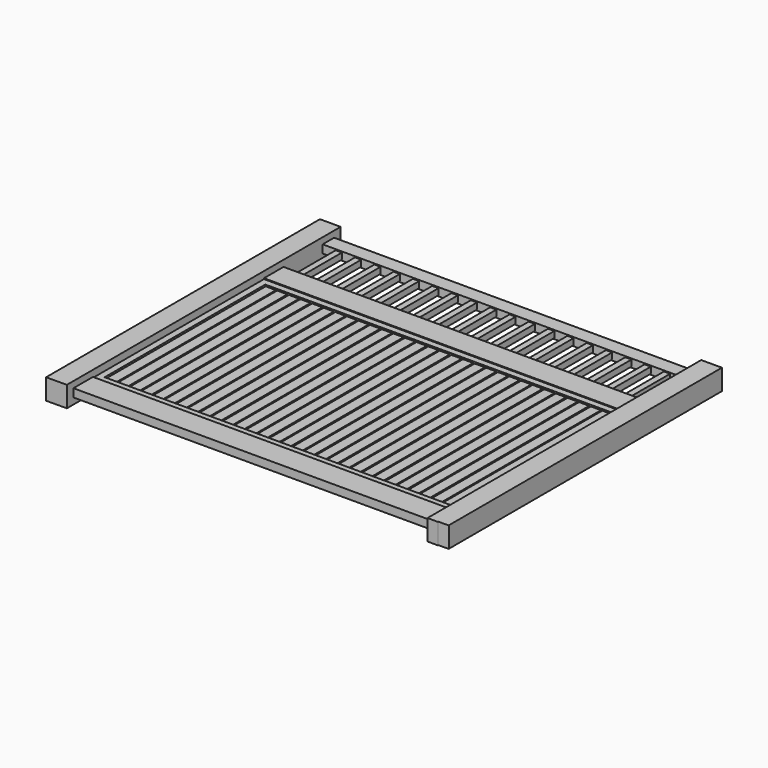
from build123d import *

# Parameters (mm, degrees)
F1_DEPTH      = 63.5
F1_DEPTH_BACK = 63.5
F2_DEPTH      = 25
F2_DEPTH_BACK = 25
F0_W          = 2213
F0_H          = 150
F0_W_2        = 40
F0_H_2        = 1232
F3_DEPTH      = 20
F3_DEPTH_BACK = 20
F0_W_3        = 38
F0_H_3        = 300
F4_DEPTH      = 19
F4_DEPTH_BACK = 19
F6_DEPTH      = 825
F6_DEPTH_BACK = 487.5


with BuildPart() as f1:
    # F0 (on Top) → F1 (new body, two sides)
    with BuildSketch(Plane.XY) as f1_sk:
        Polygon((1106.5, -1050), (1170, -1050), (1170, -1047.6227045059), align=None)
        Polygon((1106.5, -1000), (1106.5, -1050), (1170, -1047.6227045059), (1233.5, -1045.2454090118), (1233.5, 1050), (1170, 1050), (1106.5, 1050), (1106.5, 1000), (1106.5, 912), (1106.5, 612), (1106.5, 462), (1106.5, 422), (1106.5, -810), (1106.5, -850), align=None)
    extrude(amount=F1_DEPTH)
    extrude(f1_sk.sketch, amount=-F1_DEPTH_BACK)


with BuildPart() as f1b:
    # F0 (on Top) → F1, piece 2 (new body, two sides)
    with BuildSketch(Plane.XY) as f1_2_sk:
        Polygon((-1106.5, -1050), (-1106.5, -1000), (-1106.5, -850), (-1106.5, -810), (-1106.5, 422), (-1106.5, 462), (-1106.5, 612), (-1106.5, 912), (-1106.5, 1000), (-1106.5, 1050), (-1170, 1050), (-1233.5, 1050), (-1233.5, -1050.8052110672), align=None)
    extrude(amount=F1_DEPTH)
    extrude(f1_2_sk.sketch, amount=-F1_DEPTH_BACK)


with BuildPart() as f2:
    # F0 (on Top) → F2 (new body, two sides)
    with BuildSketch(Plane.XY) as f2_sk:
        Polygon((1106.5, 912), (1106.5, 1000), (-1106.5, 1000), (-1106.5, 912), (-1026.03, 912), (-988.03, 912), (-907.56, 912), (-869.56, 912), (-789.09, 912), (-751.09, 912), (-670.62, 912), (-632.62, 912), (-552.15, 912), (-514.15, 912), (-433.68, 912), (-395.68, 912), (-315.21, 912), (-277.21, 912), (-196.74, 912), (-158.74, 912), (-78.27, 912), (-40.27, 912), (40.2, 912), (78.2, 912), (158.67, 912), (196.67, 912), (277.14, 912), (315.14, 912), (395.61, 912), (433.61, 912), (514.08, 912), (552.08, 912), (632.55, 912), (670.55, 912), (751.02, 912), (789.02, 912), (869.49, 912), (907.49, 912), (987.96, 912), (1025.96, 912), align=None)
    extrude(amount=F2_DEPTH)
    extrude(f2_sk.sketch, amount=-F2_DEPTH_BACK)


with BuildPart() as f2b:
    # F0 (on Top) → F2, piece 2 (new body, two sides)
    with BuildSketch(Plane.XY) as f2_2_sk:
        Polygon((-1106.5, 462), (1106.5, 462), (1106.5, 612), (1025.96, 612), (987.96, 612), (907.49, 612), (869.49, 612), (789.02, 612), (751.02, 612), (670.55, 612), (632.55, 612), (552.08, 612), (514.08, 612), (433.61, 612), (395.61, 612), (315.14, 612), (277.14, 612), (196.67, 612), (158.67, 612), (78.2, 612), (40.2, 612), (-40.27, 612), (-78.27, 612), (-158.74, 612), (-196.74, 612), (-277.21, 612), (-315.21, 612), (-395.68, 612), (-433.68, 612), (-514.15, 612), (-552.15, 612), (-632.62, 612), (-670.62, 612), (-751.09, 612), (-789.09, 612), (-869.56, 612), (-907.56, 612), (-988.03, 612), (-1026.03, 612), (-1106.5, 612), align=None)
    extrude(amount=F2_DEPTH)
    extrude(f2_2_sk.sketch, amount=-F2_DEPTH_BACK)


with BuildPart() as f2c:
    # F0 (on Top) → F2, piece 3 (new body, two sides)
    with BuildSketch(Plane.XY) as f2_3_sk:
        with Locations((0, -925)):
            Rectangle(F0_W, F0_H)
    extrude(amount=F2_DEPTH)
    extrude(f2_3_sk.sketch, amount=-F2_DEPTH_BACK)


with BuildPart() as f3:
    # F0 (on Top) → F3 (new body, two sides)
    with BuildSketch(Plane.XY) as f3_sk:
        Polygon((1066.5, 422), (1106.5, 422), (1106.5, 462), (-1106.5, 462), (-1106.5, 422), (-1066.5, 422), align=None)
        with Locations((1086.5, -194)):
            Rectangle(F0_W_2, F0_H_2)
        Polygon((-1106.5, -850), (1106.5, -850), (1106.5, -810), (1066.5, -810), (-1066.5, -810), (-1106.5, -810), align=None)
        with Locations((-1086.5, -194)):
            Rectangle(F0_W_2, F0_H_2)
    extrude(amount=F3_DEPTH)
    extrude(f3_sk.sketch, amount=-F3_DEPTH_BACK)

    # F5 (on Front) → F6 (join, two sides)
    with BuildSketch(Plane.XZ) as f6_sk:
        Polygon((-992.4924378616, -11), (-931.2006182523, -11), (-927.5, -7.6376459808), (-927.5, 7.3770178367), (-930.9458671252, 11), (-993.3938319101, 11), (-997.3938319101, 8), (-1001.3938319101, 11), (-1063.7911305095, 11), (-1067.5, 7.6467497703), (-1067.5, -8.3163099906), (-1063.2812551709, -11), (-1000.4924378616, -11), (-996.4924378616, -8), align=None)
        Polygon((-920.7812551709, -11), (-857.9924378616, -11), (-853.9924378616, -8), (-849.9924378616, -11), (-788.7006182523, -11), (-785, -7.6376459808), (-785, 7.3770178367), (-788.4458671252, 11), (-850.8938319101, 11), (-854.8938319101, 8), (-858.8938319101, 11), (-921.2911305095, 11), (-925, 7.6467497703), (-925, -8.3163099906), align=None)
        Polygon((-778.2812551709, -11), (-715.4924378616, -11), (-711.4924378616, -8), (-707.4924378616, -11), (-646.2006182523, -11), (-642.5, -7.6376459808), (-642.5, 7.3770178367), (-645.9458671252, 11), (-708.3938319101, 11), (-712.3938319101, 8), (-716.3938319101, 11), (-778.7911305095, 11), (-782.5, 7.6467497703), (-782.5, -8.3163099906), align=None)
        Polygon((-635.7812551709, -11), (-572.9924378616, -11), (-568.9924378616, -8), (-564.9924378616, -11), (-503.7006182523, -11), (-500, -7.6376459808), (-500, 7.3770178367), (-503.4458671252, 11), (-565.8938319101, 11), (-569.8938319101, 8), (-573.8938319101, 11), (-636.2911305095, 11), (-640, 7.6467497703), (-640, -8.3163099906), align=None)
        Polygon((-493.2812551709, -11), (-430.4924378616, -11), (-426.4924378616, -8), (-422.4924378616, -11), (-361.2006182523, -11), (-357.5, -7.6376459808), (-357.5, 7.3770178367), (-360.9458671252, 11), (-423.3938319101, 11), (-427.3938319101, 8), (-431.3938319101, 11), (-493.7911305095, 11), (-497.5, 7.6467497703), (-497.5, -8.3163099906), align=None)
        Polygon((-350.7812551709, -11), (-287.9924378616, -11), (-283.9924378616, -8), (-279.9924378616, -11), (-218.7006182523, -11), (-215, -7.6376459808), (-215, 7.3770178367), (-218.4458671252, 11), (-280.8938319101, 11), (-284.8938319101, 8), (-288.8938319101, 11), (-351.2911305095, 11), (-355, 7.6467497703), (-355, -8.3163099906), align=None)
        Polygon((-208.2812551709, -11), (-145.4924378616, -11), (-141.4924378616, -8), (-137.4924378616, -11), (-76.2006182523, -11), (-72.5, -7.6376459808), (-72.5, 7.3770178367), (-75.9458671252, 11), (-138.3938319101, 11), (-142.3938319101, 8), (-146.3938319101, 11), (-208.7911305095, 11), (-212.5, 7.6467497703), (-212.5, -8.3163099906), align=None)
        Polygon((-65.7812551709, -11), (-2.9924378616, -11), (1.0075621384, -8), (5.0075621384, -11), (66.2993817477, -11), (70, -7.6376459808), (70, 7.3770178367), (66.5541328748, 11), (4.1061680899, 11), (0.1061680899, 8), (-3.8938319101, 11), (-66.2911305095, 11), (-70, 7.6467497703), (-70, -8.3163099906), align=None)
        Polygon((76.7187448291, -11), (139.5075621384, -11), (143.5075621384, -8), (147.5075621384, -11), (208.7993817477, -11), (212.5, -7.6376459808), (212.5, 7.3770178367), (209.0541328748, 11), (146.6061680899, 11), (142.6061680899, 8), (138.6061680899, 11), (76.2088694905, 11), (72.5, 7.6467497703), (72.5, -8.3163099906), align=None)
        Polygon((219.2187448291, -11), (282.0075621384, -11), (286.0075621384, -8), (290.0075621384, -11), (351.2993817477, -11), (355, -7.6376459808), (355, 7.3770178367), (351.5541328748, 11), (289.1061680899, 11), (285.1061680899, 8), (281.1061680899, 11), (218.7088694905, 11), (215, 7.6467497703), (215, -8.3163099906), align=None)
        Polygon((361.7187448291, -11), (424.5075621384, -11), (428.5075621384, -8), (432.5075621384, -11), (493.7993817477, -11), (497.5, -7.6376459808), (497.5, 7.3770178367), (494.0541328748, 11), (431.6061680899, 11), (427.6061680899, 8), (423.6061680899, 11), (361.2088694905, 11), (357.5, 7.6467497703), (357.5, -8.3163099906), align=None)
        Polygon((504.2187448291, -11), (567.0075621384, -11), (571.0075621384, -8), (575.0075621384, -11), (636.2993817477, -11), (640, -7.6376459808), (640, 7.3770178367), (636.5541328748, 11), (574.1061680899, 11), (570.1061680899, 8), (566.1061680899, 11), (503.7088694905, 11), (500, 7.6467497703), (500, -8.3163099906), align=None)
        Polygon((646.7187448291, -11), (709.5075621384, -11), (713.5075621384, -8), (717.5075621384, -11), (778.7993817477, -11), (782.5, -7.6376459808), (782.5, 7.3770178367), (779.0541328748, 11), (716.6061680899, 11), (712.6061680899, 8), (708.6061680899, 11), (646.2088694905, 11), (642.5, 7.6467497703), (642.5, -8.3163099906), align=None)
        Polygon((789.2187448291, -11), (852.0075621384, -11), (856.0075621384, -8), (860.0075621384, -11), (921.2993817477, -11), (925, -7.6376459808), (925, 7.3770178367), (921.5541328748, 11), (859.1061680899, 11), (855.1061680899, 8), (851.1061680899, 11), (788.7088694905, 11), (785, 7.6467497703), (785, -8.3163099906), align=None)
        Polygon((931.7187448291, -11), (994.5075621384, -11), (998.5075621384, -8), (1002.5075621384, -11), (1063.7993817477, -11), (1067.5, -7.6376459808), (1067.5, 7.3770178367), (1064.0541328748, 11), (1001.6061680899, 11), (997.6061680899, 8), (993.6061680899, 11), (931.2088694905, 11), (927.5, 7.6467497703), (927.5, -8.3163099906), align=None)
    extrude(amount=F6_DEPTH)
    extrude(f6_sk.sketch, amount=-F6_DEPTH_BACK)


with BuildPart() as f4:
    # F0 (on Top) → F4 (new body, two sides)
    with BuildSketch(Plane.XY) as f4_sk:
        with Locations((-1007.03, 762)):
            Rectangle(F0_W_3, F0_H_3)
    extrude(amount=F4_DEPTH)
    extrude(f4_sk.sketch, amount=-F4_DEPTH_BACK)


with BuildPart() as f4b:
    # F0 (on Top) → F4, piece 2 (new body, two sides)
    with BuildSketch(Plane.XY) as f4_2_sk:
        with Locations((-888.56, 762)):
            Rectangle(F0_W_3, F0_H_3)
    extrude(amount=F4_DEPTH)
    extrude(f4_2_sk.sketch, amount=-F4_DEPTH_BACK)


with BuildPart() as f4c:
    # F0 (on Top) → F4, piece 3 (new body, two sides)
    with BuildSketch(Plane.XY) as f4_3_sk:
        with Locations((-770.09, 762)):
            Rectangle(F0_W_3, F0_H_3)
    extrude(amount=F4_DEPTH)
    extrude(f4_3_sk.sketch, amount=-F4_DEPTH_BACK)


with BuildPart() as f4d:
    # F0 (on Top) → F4, piece 4 (new body, two sides)
    with BuildSketch(Plane.XY) as f4_4_sk:
        with Locations((-651.62, 762)):
            Rectangle(F0_W_3, F0_H_3)
    extrude(amount=F4_DEPTH)
    extrude(f4_4_sk.sketch, amount=-F4_DEPTH_BACK)


with BuildPart() as f4e:
    # F0 (on Top) → F4, piece 5 (new body, two sides)
    with BuildSketch(Plane.XY) as f4_5_sk:
        with Locations((-533.15, 762)):
            Rectangle(F0_W_3, F0_H_3)
    extrude(amount=F4_DEPTH)
    extrude(f4_5_sk.sketch, amount=-F4_DEPTH_BACK)


with BuildPart() as f4f:
    # F0 (on Top) → F4, piece 6 (new body, two sides)
    with BuildSketch(Plane.XY) as f4_6_sk:
        with Locations((-414.68, 762)):
            Rectangle(F0_W_3, F0_H_3)
    extrude(amount=F4_DEPTH)
    extrude(f4_6_sk.sketch, amount=-F4_DEPTH_BACK)


with BuildPart() as f4g:
    # F0 (on Top) → F4, piece 7 (new body, two sides)
    with BuildSketch(Plane.XY) as f4_7_sk:
        with Locations((-296.21, 762)):
            Rectangle(F0_W_3, F0_H_3)
    extrude(amount=F4_DEPTH)
    extrude(f4_7_sk.sketch, amount=-F4_DEPTH_BACK)


with BuildPart() as f4h:
    # F0 (on Top) → F4, piece 8 (new body, two sides)
    with BuildSketch(Plane.XY) as f4_8_sk:
        with Locations((-177.74, 762)):
            Rectangle(F0_W_3, F0_H_3)
    extrude(amount=F4_DEPTH)
    extrude(f4_8_sk.sketch, amount=-F4_DEPTH_BACK)


with BuildPart() as f4i:
    # F0 (on Top) → F4, piece 9 (new body, two sides)
    with BuildSketch(Plane.XY) as f4_9_sk:
        with Locations((-59.27, 762)):
            Rectangle(F0_W_3, F0_H_3)
    extrude(amount=F4_DEPTH)
    extrude(f4_9_sk.sketch, amount=-F4_DEPTH_BACK)


with BuildPart() as f4j:
    # F0 (on Top) → F4, piece 10 (new body, two sides)
    with BuildSketch(Plane.XY) as f4_10_sk:
        with Locations((59.2, 762)):
            Rectangle(F0_W_3, F0_H_3)
    extrude(amount=F4_DEPTH)
    extrude(f4_10_sk.sketch, amount=-F4_DEPTH_BACK)


with BuildPart() as f4k:
    # F0 (on Top) → F4, piece 11 (new body, two sides)
    with BuildSketch(Plane.XY) as f4_11_sk:
        with Locations((177.67, 762)):
            Rectangle(F0_W_3, F0_H_3)
    extrude(amount=F4_DEPTH)
    extrude(f4_11_sk.sketch, amount=-F4_DEPTH_BACK)


with BuildPart() as f4l:
    # F0 (on Top) → F4, piece 12 (new body, two sides)
    with BuildSketch(Plane.XY) as f4_12_sk:
        with Locations((296.14, 762)):
            Rectangle(F0_W_3, F0_H_3)
    extrude(amount=F4_DEPTH)
    extrude(f4_12_sk.sketch, amount=-F4_DEPTH_BACK)


with BuildPart() as f4m:
    # F0 (on Top) → F4, piece 13 (new body, two sides)
    with BuildSketch(Plane.XY) as f4_13_sk:
        with Locations((414.61, 762)):
            Rectangle(F0_W_3, F0_H_3)
    extrude(amount=F4_DEPTH)
    extrude(f4_13_sk.sketch, amount=-F4_DEPTH_BACK)


with BuildPart() as f4n:
    # F0 (on Top) → F4, piece 14 (new body, two sides)
    with BuildSketch(Plane.XY) as f4_14_sk:
        with Locations((533.08, 762)):
            Rectangle(F0_W_3, F0_H_3)
    extrude(amount=F4_DEPTH)
    extrude(f4_14_sk.sketch, amount=-F4_DEPTH_BACK)


with BuildPart() as f4o:
    # F0 (on Top) → F4, piece 15 (new body, two sides)
    with BuildSketch(Plane.XY) as f4_15_sk:
        with Locations((651.55, 762)):
            Rectangle(F0_W_3, F0_H_3)
    extrude(amount=F4_DEPTH)
    extrude(f4_15_sk.sketch, amount=-F4_DEPTH_BACK)


with BuildPart() as f4p:
    # F0 (on Top) → F4, piece 16 (new body, two sides)
    with BuildSketch(Plane.XY) as f4_16_sk:
        with Locations((770.02, 762)):
            Rectangle(F0_W_3, F0_H_3)
    extrude(amount=F4_DEPTH)
    extrude(f4_16_sk.sketch, amount=-F4_DEPTH_BACK)


with BuildPart() as f4q:
    # F0 (on Top) → F4, piece 17 (new body, two sides)
    with BuildSketch(Plane.XY) as f4_17_sk:
        with Locations((888.49, 762)):
            Rectangle(F0_W_3, F0_H_3)
    extrude(amount=F4_DEPTH)
    extrude(f4_17_sk.sketch, amount=-F4_DEPTH_BACK)


with BuildPart() as f4r:
    # F0 (on Top) → F4, piece 18 (new body, two sides)
    with BuildSketch(Plane.XY) as f4_18_sk:
        with Locations((1006.96, 762)):
            Rectangle(F0_W_3, F0_H_3)
    extrude(amount=F4_DEPTH)
    extrude(f4_18_sk.sketch, amount=-F4_DEPTH_BACK)


solid = Compound([f1.part, f1b.part, f2.part, f2b.part, f2c.part, f3.part, f4.part, f4b.part, f4c.part, f4d.part, f4e.part, f4f.part, f4g.part, f4h.part, f4i.part, f4j.part, f4k.part, f4l.part, f4m.part, f4n.part, f4o.part, f4p.part, f4q.part, f4r.part])
